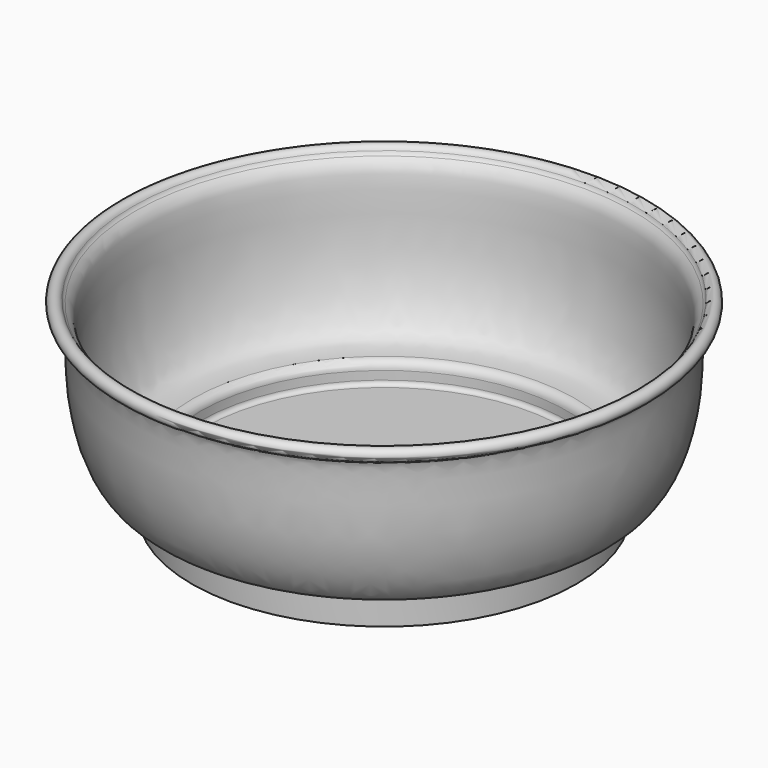
from build123d import *

# Parameters (mm, degrees)
F2_R     = 1
F3_R     = 45
F3_R_2   = 43
F4_DEPTH = 2


# Not quite as in the source:
# - ends of sketch curves that miss each other by under 0.0002 mm in the source are joined
# - the dataset's text gives a spline's control points without its knots; the knots are read off the source's solid


with BuildPart() as f1:
    # F0 (on Front) → F1 (revolve)
    with BuildSketch(Plane.XZ):
        with BuildLine():
            Line((0, 2), (0, 0))
            Line((0, 0), (45, 0))
            Line((45, 0), (45, 4.1077052209))
            ThreePointArc((45, 4.1077052209), (45.251607634, 4.770961481), (45.8798177332, 5.1004570644))
            add(Edge.make_bspline(
                [(59.117932503, 39.1061978883), (58.9984398686, 38.9167118255), (57.961379378, 36.7467385449), (59.1133721589, 22.9753032204), (53.6275212518, 6.4619991243), (47.9608297571, 5.3523838112), (45.8798177332, 5.1004570644)],
                knots=[0.079529872, 0.079529872, 0.079529872, 0.079529872, 0.1164806675, 0.435781553, 0.7789347917, 0.9727324769, 0.9727324769, 0.9727324769, 0.9727324769], degree=3))
            ThreePointArc((59.117932503, 39.1061978883), (59.7042053248, 39.7061118302), (60.4849287438, 40.0128421715))
            ThreePointArc((60.4849287438, 40.0128421715), (61.4445872468, 42.4401309197), (58.8691826, 42.0159069052))
            ThreePointArc((58.8691826, 42.0159069052), (58.643182834, 41.577442369), (58.31674753, 41.2076237072))
            add(Edge.make_bspline(
                [(58.31674753, 41.2076237072), (58.3148397341, 41.2059420359), (58.1329946532, 41.0449587485), (57.8276969018, 40.7452853769), (57.4453837385, 40.220259631), (57.1893214461, 39.771564073), (56.9743902421, 39.277445408), (56.8043597407, 38.7424234539), (56.680003708, 38.203859582), (56.5520410764, 37.4591588813), (56.4452689195, 36.4663757584), (56.3674656809, 35.155302403), (56.3050858948, 33.2523114152), (56.2634042278, 30.6110777497), (56.1735934989, 27.7415742893), (56.018450433, 25.3953023971), (55.8477339812, 23.6368985798), (55.6092469781, 21.8895853556), (55.2036356572, 19.5864432025), (54.539773, 16.8097339131), (53.5203746444, 13.7898979021), (52.5184171783, 11.6646836577), (51.6611889381, 10.2810715096), (51.1154343385, 9.5653431356), (50.6822443153, 9.0894464967), (50.3647724491, 8.7843429997), (50.0474792797, 8.5214792406), (49.6165481094, 8.2146567762), (49.059056291, 7.9027315772), (48.0980536701, 7.5169322584), (46.7280561328, 7.2056808972), (45.4526028209, 7.0623561488), (44.7798504425, 6.9878504754)],
                knots=[0.0309186802, 0.0309186802, 0.0309186802, 0.0309186802, 0.03125, 0.0625, 0.078125, 0.09375, 0.109375, 0.125, 0.140625, 0.15625, 0.1875, 0.21875, 0.25, 0.3125, 0.375, 0.40625, 0.4375, 0.46875, 0.5, 0.5625, 0.625, 0.6875, 0.71875, 0.75, 0.765625, 0.78125, 0.796875, 0.8125, 0.84375, 0.875, 0.9375, 1, 1, 1, 1], degree=3))
            ThreePointArc((44.7798504425, 6.9878504754), (43.5099827366, 6.3341112085), (42.9999989595, 5))
            Line((42.9999989595, 5), (42.9999994798, 2))
            Line((42.9999994798, 2), (0, 2))
        make_face()
    revolve(axis=Axis((0, 0, 20.8975244313), (0, 0, 1)))

    # F2
    f2_edges = [f1.edges().sort_by_distance(p)[0] for p in [
        (-42.999999, 0, 2),
    ]]
    fillet(f2_edges, radius=F2_R)

    # F3 (on face) → F4 (join)
    with BuildSketch(Plane(origin=(0, 0, 0), x_dir=(1, 0, 0), z_dir=(0, 0, -1))):
        Circle(F3_R)
        Circle(F3_R_2, mode=Mode.SUBTRACT)
    extrude(amount=F4_DEPTH)


solid = f1.part
